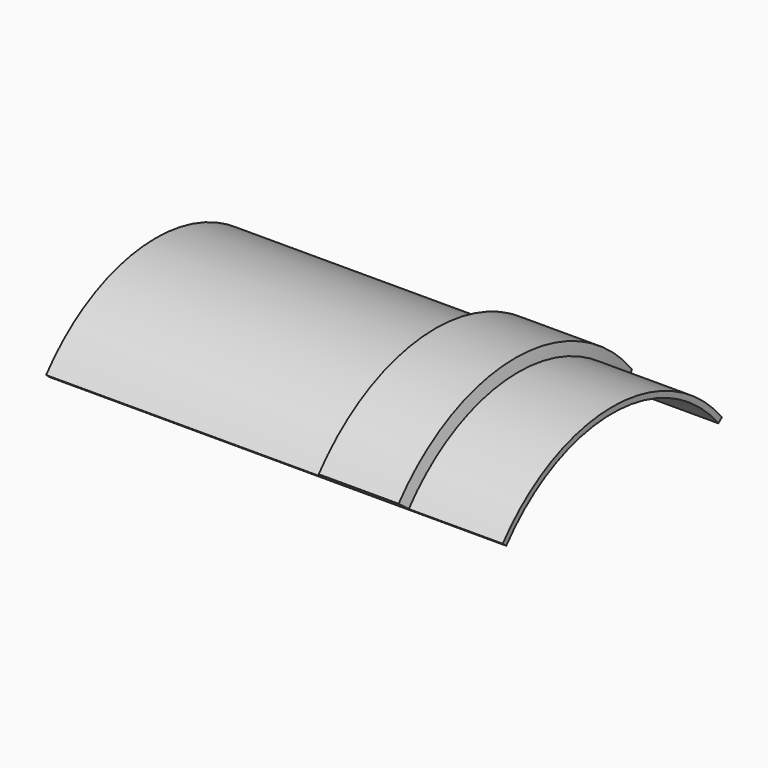
from build123d import *

# Parameters (mm, degrees)
F1_DEPTH = 127


# Not quite as in the source:
# - a feature of the source that left no trace in its solid (it failed there, or was rolled back) is left out


with BuildPart() as f1:
    # F0 (on Right) → F1 (new body, symmetric)
    with BuildSketch(Plane.YZ):
        with BuildLine():
            ThreePointArc((0, 34.925), (40.7978992511, 25.7523970758), (73.743601134, 0))
            Line((73.743601134, 0), (76.2, 2.011648481))
            ThreePointArc((76.2, 2.011648481), (42.1568770053, 28.6218577331), (0, 38.1))
            ThreePointArc((0, 38.1), (-42.1568770053, 28.6218577331), (-76.2, 2.011648481))
            Line((-76.2, 2.011648481), (-73.743601134, 0))
            ThreePointArc((-73.743601134, 0), (-40.7978992511, 25.7523970758), (0, 34.925))
        make_face()
    extrude(amount=F1_DEPTH, both=True)


with BuildPart() as f5:
    # F5: sweep along a path in F4
    with BuildLine(Plane.YZ.offset(75.5772160579)) as f5_path:
        ThreePointArc((-76.2, 2.011648481), (0, 38.1), (76.2, 2.011648481))
    # F2 (on face) → F5 (sweep)
    with BuildSketch(Plane(origin=(0, -29.6033643096, -36.1482988732), x_dir=(1, 0, 0), z_dir=(0, -0.6335900728, -0.7736689342))):
        Polygon((73.025, 66.5781332912), (50.8, 66.5781332912), (28.575, 66.5781332912), (26.8735226281, 60.2281332912), (74.7264773719, 60.2281332912), align=None)
    sweep(path=f5_path.line)


solid = Compound([f1.part, f5.part])
